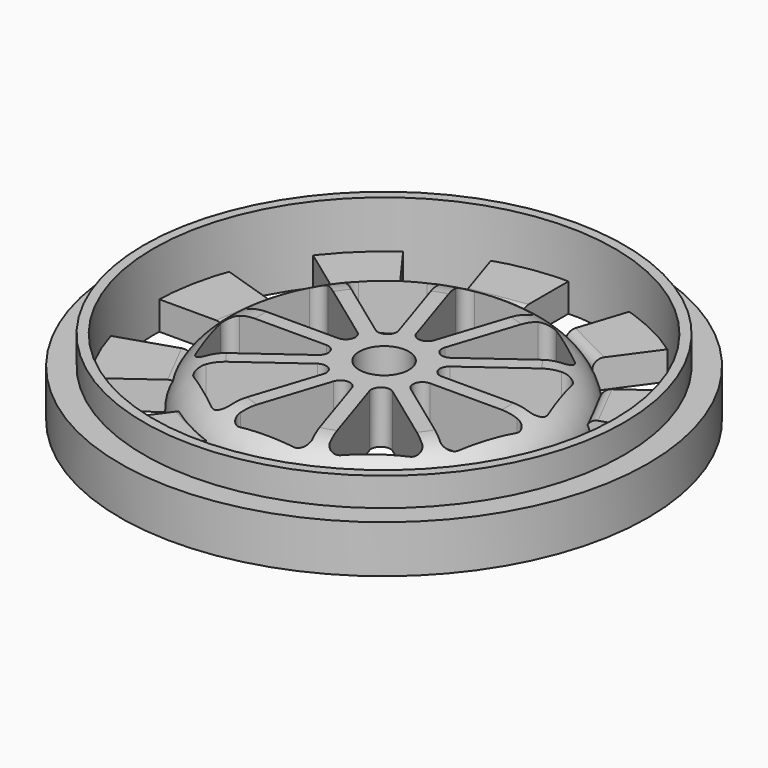
from build123d import *

# Parameters (mm, degrees)
F0_W      = 2.5
F0_H      = 5
F2_R      = 18
F2_R_2    = 1.25
F3_DEPTH  = 5.5
F5_DEPTH  = 3
F6_R      = 1
F7_R      = 1
F7_2_R    = 1
F7_3_R    = 1
F7_4_R    = 1
F7_5_R    = 1
F7_6_R    = 1
F7_7_R    = 1
F7_8_R    = 1
F7_9_R    = 1
F7_10_R   = 1
F8_R      = 1
F9_R      = 2.6095979765
F9_R_2    = 1.25
F10_DEPTH = 3


# Not quite as in the source:
# - a fillet or chamfer that OpenCascade refuses, or shapes differently, is made with other operations: its cross-section is extruded or revolved along the edge and cut away or added


with BuildPart() as f1:
    # F0 (on Front) → F1 (revolve)
    with BuildSketch(Plane.XZ):
        Polygon((24.2499966236, 8.000213087), (24.2499966236, 0.000213087), (25.2499966236, 0.000213087), (25.2499966236, 5.000213087), (25.2499966236, 8.000213087), align=None)
        with Locations((26.4999966236, 2.500213087)):
            Rectangle(F0_W, F0_H)
    revolve(axis=Axis((0, 0, 5.9403805062), (0, 0, -1)))


with BuildPart() as f3:
    # F2 (on Top) → F3 (new body)
    with BuildSketch(Plane.XY):
        Circle(F2_R)
        Polygon((-15.9813384329, -0.7725424859), (-2.3776412907, -0.7725424859), (-13.3832634651, -8.7685950428), align=None, mode=Mode.SUBTRACT)
        Polygon((-12.4750853051, -10.0185950428), (-1.4694631307, -2.0225424859), (-5.673236734, -14.9604272987), align=None, mode=Mode.SUBTRACT)
        Polygon((-4.2037736033, -15.4378848128), (0, -2.5), (4.2037736033, -15.4378848128), align=None, mode=Mode.SUBTRACT)
        Polygon((5.673236734, -14.9604272987), (1.4694631307, -2.0225424859), (12.4750853051, -10.0185950428), align=None, mode=Mode.SUBTRACT)
        Polygon((13.3832634651, -8.7685950428), (2.3776412907, -0.7725424859), (15.9813384329, -0.7725424859), align=None, mode=Mode.SUBTRACT)
        Polygon((-13.3832634651, 8.7685950428), (-2.3776412907, 0.7725424859), (-15.9813384329, 0.7725424859), align=None, mode=Mode.SUBTRACT)
        Polygon((-5.673236734, 14.9604272987), (-1.4694631307, 2.0225424859), (-12.4750853051, 10.0185950428), align=None, mode=Mode.SUBTRACT)
        with BuildLine():
            ThreePointArc((2.3776412907, 0.7725424859), (2.4692208515, 0.3910861626), (2.5, 0))
            ThreePointArc((2.5, 0), (2.4692208515, -0.3910861626), (2.3776412907, -0.7725424859))
            ThreePointArc((2.3776412907, -0.7725424859), (2.0225424859, -1.4694631307), (1.4694631307, -2.0225424859))
            ThreePointArc((1.4694631307, -2.0225424859), (0.7725424859, -2.3776412907), (0, -2.5))
            ThreePointArc((0, -2.5), (-0.7725424859, -2.3776412907), (-1.4694631307, -2.0225424859))
            ThreePointArc((-1.4694631307, -2.0225424859), (-2.0225424859, -1.4694631307), (-2.3776412907, -0.7725424859))
            ThreePointArc((-2.3776412907, -0.7725424859), (-2.5, 0), (-2.3776412907, 0.7725424859))
            ThreePointArc((-2.3776412907, 0.7725424859), (-2.0225424859, 1.4694631307), (-1.4694631307, 2.0225424859))
            ThreePointArc((-1.4694631307, 2.0225424859), (-0.7725424859, 2.3776412907), (0, 2.5))
            ThreePointArc((0, 2.5), (0.7725424859, 2.3776412907), (1.4694631307, 2.0225424859))
            ThreePointArc((1.4694631307, 2.0225424859), (2.0225424859, 1.4694631307), (2.3776412907, 0.7725424859))
        make_face(mode=Mode.SUBTRACT)
        Polygon((4.2037736033, 15.4378848128), (0, 2.5), (-4.2037736033, 15.4378848128), align=None, mode=Mode.SUBTRACT)
        Polygon((12.4750853051, 10.0185950428), (1.4694631307, 2.0225424859), (5.673236734, 14.9604272987), align=None, mode=Mode.SUBTRACT)
        Polygon((15.9813384329, 0.7725424859), (2.3776412907, 0.7725424859), (13.3832634651, 8.7685950428), align=None, mode=Mode.SUBTRACT)
        with BuildLine():
            ThreePointArc((2.3776412907, -0.7725424859), (2.4692208515, -0.3910861626), (2.5, 0))
            ThreePointArc((2.5, 0), (2.4692208515, 0.3910861626), (2.3776412907, 0.7725424859))
            ThreePointArc((2.3776412907, 0.7725424859), (2.0225424859, 1.4694631307), (1.4694631307, 2.0225424859))
            ThreePointArc((1.4694631307, 2.0225424859), (0.7725424859, 2.3776412907), (0, 2.5))
            ThreePointArc((0, 2.5), (-0.7725424859, 2.3776412907), (-1.4694631307, 2.0225424859))
            ThreePointArc((-1.4694631307, 2.0225424859), (-2.0225424859, 1.4694631307), (-2.3776412907, 0.7725424859))
            ThreePointArc((-2.3776412907, 0.7725424859), (-2.5, 0), (-2.3776412907, -0.7725424859))
            ThreePointArc((-2.3776412907, -0.7725424859), (-2.0225424859, -1.4694631307), (-1.4694631307, -2.0225424859))
            ThreePointArc((-1.4694631307, -2.0225424859), (-0.7725424859, -2.3776412907), (0, -2.5))
            ThreePointArc((0, -2.5), (0.7725424859, -2.3776412907), (1.4694631307, -2.0225424859))
            ThreePointArc((1.4694631307, -2.0225424859), (2.0225424859, -1.4694631307), (2.3776412907, -0.7725424859))
        make_face()
        Circle(F2_R_2, mode=Mode.SUBTRACT)
    extrude(amount=F3_DEPTH)

    # F6
    f6_edges = [f3.edges().sort_by_distance(p)[0] for p in [
        (-5.673237, 14.960427, 2.75),
        (4.203774, 15.437885, 2.75),
        (12.475085, 10.018595, 2.75),
        (15.981338, 0.772542, 2.75),
        (13.383263, -8.768595, 2.75),
        (5.673237, -14.960427, 2.75),
        (-4.203774, -15.437885, 2.75),
        (-12.475085, -10.018595, 2.75),
        (-15.981338, -0.772542, 2.75),
        (-13.383263, 8.768595, 2.75),
        (13.383263, 8.768595, 2.75),
        (5.673237, 14.960427, 2.75),
        (-4.203774, 15.437885, 2.75),
        (-12.475085, 10.018595, 2.75),
        (-15.981338, 0.772542, 2.75),
        (-13.383263, -8.768595, 2.75),
        (-5.673237, -14.960427, 2.75),
        (4.203774, -15.437885, 2.75),
        (12.475085, -10.018595, 2.75),
        (15.981338, -0.772542, 2.75),
    ]]
    fillet(f6_edges, radius=F6_R)

    # F8
    f8_edges = [f3.edges().sort_by_distance(p)[0] for p in [
        (-2.377641, 0.772542, 2.75),
        (-2.377641, -0.772542, 2.75),
        (-1.469463, -2.022542, 2.75),
        (0, -2.5, 2.75),
        (1.469463, -2.022542, 2.75),
        (2.377641, -0.772542, 2.75),
        (2.377641, 0.772542, 2.75),
        (1.469463, 2.022542, 2.75),
        (0, 2.5, 2.75),
        (-1.469463, 2.022542, 2.75),
    ]]
    fillet(f8_edges, radius=F8_R)

    # F9 (on face) → F10 (cut)
    with BuildSketch(Plane.XY.offset(5.5)):
        Circle(F9_R)
        Circle(F9_R_2, mode=Mode.SUBTRACT)
    extrude(amount=-F10_DEPTH, mode=Mode.SUBTRACT)

    # F11: fillet of radius 5 on 1 edges, made by hand

    # F11_s1 → F11_t2 (revolve, cut)
    with BuildSketch(Plane.XZ):
        with BuildLine():
            ThreePointArc((18, 0.5), (16.5355339059, 4.0355339059), (13, 5.5))
            Line((13, 5.5), (18, 5.5))
            Line((18, 5.5), (18, 0.5))
        make_face()
    revolve(axis=Axis((0, 0, 5.5), (0, 0, 1)), mode=Mode.SUBTRACT)


with BuildPart() as f5:
    # F4 (on Top) → F5 (new body)
    with BuildSketch(Plane.XY):
        Polygon((-13.955543153, 10.889295602), (-10.139295602, 14.705543153), (-14.8415776204, 21.177679108), (-20.427679108, 15.5915776204), align=None)
    extrude(amount=F5_DEPTH)

    # F7#2
    f7_2_edges = [f5.edges().sort_by_distance(p)[0] for p in [
        (-12.047419, 12.797419, 3),
    ]]
    fillet(f7_2_edges, radius=F7_2_R)


with BuildPart() as f5b:
    # F4 (on Top) → F5, piece 2 (new body)
    with BuildSketch(Plane.XY):
        Polygon((-5.330543153, 17.1557249061), (0, 18), (0, 26), (-7.802679108, 24.7641770365), align=None)
    extrude(amount=F5_DEPTH)

    # F7
    f7_edges = [f5b.edges().sort_by_distance(p)[0] for p in [
        (-2.665272, 17.577862, 3),
    ]]
    fillet(f7_edges, radius=F7_R)


with BuildPart() as f5c:
    # F4 (on Top) → F5, piece 3 (new body)
    with BuildSketch(Plane.XY):
        Polygon((5.330543153, 17.1557249061), (10.139295602, 14.705543153), (14.8415776204, 21.177679108), (7.802679108, 24.7641770365), align=None)
    extrude(amount=F5_DEPTH)

    # F7#10
    f7_10_edges = [f5c.edges().sort_by_distance(p)[0] for p in [
        (7.734919, 15.930634, 3),
    ]]
    fillet(f7_10_edges, radius=F7_10_R)


with BuildPart() as f5d:
    # F4 (on Top) → F5, piece 4 (new body)
    with BuildSketch(Plane.XY):
        Polygon((13.955543153, 10.889295602), (16.4057249061, 6.080543153), (24.0141770365, 8.552679108), (20.427679108, 15.5915776204), align=None)
    extrude(amount=F5_DEPTH)

    # F7#9
    f7_9_edges = [f5d.edges().sort_by_distance(p)[0] for p in [
        (15.180634, 8.484919, 3),
    ]]
    fillet(f7_9_edges, radius=F7_9_R)


with BuildPart() as f5e:
    # F4 (on Top) → F5, piece 5 (new body)
    with BuildSketch(Plane.XY):
        Polygon((17.25, 0.75), (16.4057249061, -4.580543153), (24.0141770365, -7.052679108), (25.25, 0.75), align=None)
    extrude(amount=F5_DEPTH)

    # F7#8
    f7_8_edges = [f5e.edges().sort_by_distance(p)[0] for p in [
        (16.827862, -1.915272, 3),
    ]]
    fillet(f7_8_edges, radius=F7_8_R)


with BuildPart() as f5f:
    # F4 (on Top) → F5, piece 6 (new body)
    with BuildSketch(Plane.XY):
        Polygon((13.955543153, -9.389295602), (10.139295602, -13.205543153), (14.8415776204, -19.677679108), (20.427679108, -14.0915776204), align=None)
    extrude(amount=F5_DEPTH)

    # F7#7
    f7_7_edges = [f5f.edges().sort_by_distance(p)[0] for p in [
        (12.047419, -11.297419, 3),
    ]]
    fillet(f7_7_edges, radius=F7_7_R)


with BuildPart() as f5g:
    # F4 (on Top) → F5, piece 7 (new body)
    with BuildSketch(Plane.XY):
        Polygon((5.330543153, -15.6557249061), (0, -16.5), (0, -24.5), (7.802679108, -23.2641770365), align=None)
    extrude(amount=F5_DEPTH)

    # F7#6
    f7_6_edges = [f5g.edges().sort_by_distance(p)[0] for p in [
        (2.665272, -16.077862, 3),
    ]]
    fillet(f7_6_edges, radius=F7_6_R)


with BuildPart() as f5h:
    # F4 (on Top) → F5, piece 8 (new body)
    with BuildSketch(Plane.XY):
        Polygon((-5.330543153, -15.6557249061), (-10.139295602, -13.205543153), (-14.8415776204, -19.677679108), (-7.802679108, -23.2641770365), align=None)
    extrude(amount=F5_DEPTH)

    # F7#5
    f7_5_edges = [f5h.edges().sort_by_distance(p)[0] for p in [
        (-7.734919, -14.430634, 3),
    ]]
    fillet(f7_5_edges, radius=F7_5_R)


with BuildPart() as f5i:
    # F4 (on Top) → F5, piece 9 (new body)
    with BuildSketch(Plane.XY):
        Polygon((-13.955543153, -9.389295602), (-16.4057249061, -4.580543153), (-24.0141770365, -7.052679108), (-20.427679108, -14.0915776204), align=None)
    extrude(amount=F5_DEPTH)

    # F7#4
    f7_4_edges = [f5i.edges().sort_by_distance(p)[0] for p in [
        (-15.180634, -6.984919, 3),
    ]]
    fillet(f7_4_edges, radius=F7_4_R)


with BuildPart() as f5j:
    # F4 (on Top) → F5, piece 10 (new body)
    with BuildSketch(Plane.XY):
        Polygon((-17.25, 0.75), (-16.4057249061, 6.080543153), (-24.0141770365, 8.552679108), (-25.25, 0.75), align=None)
    extrude(amount=F5_DEPTH)

    # F7#3
    f7_3_edges = [f5j.edges().sort_by_distance(p)[0] for p in [
        (-16.827862, 3.415272, 3),
    ]]
    fillet(f7_3_edges, radius=F7_3_R)


solid = Compound([f1.part, f3.part, f5.part, f5b.part, f5c.part, f5d.part, f5e.part, f5f.part, f5g.part, f5h.part, f5i.part, f5j.part])
